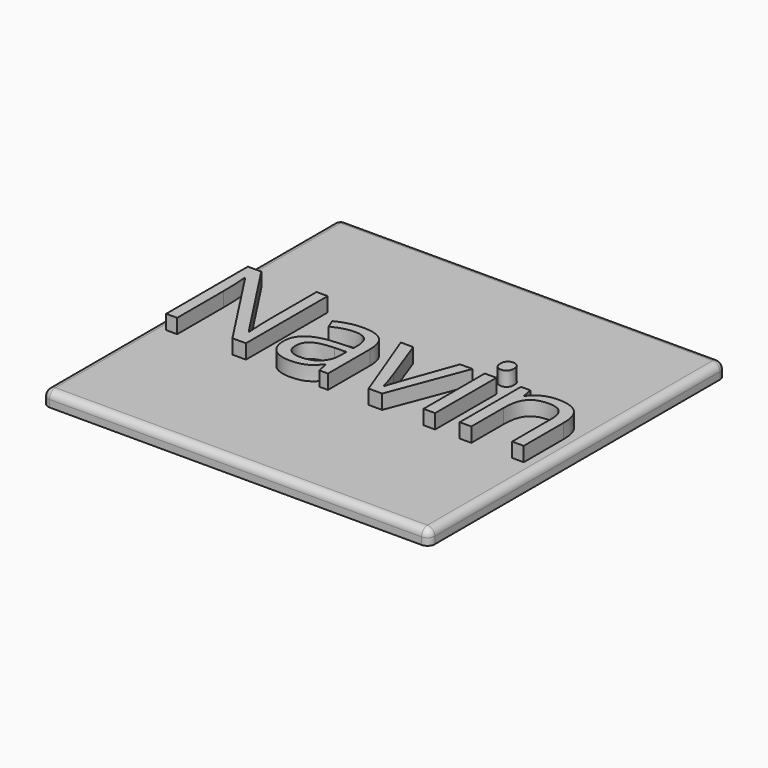
from build123d import *

# Parameters (mm, degrees)
F0_W         = 133.965395391
F0_H         = 128.5353191197
F1_DEPTH     = 5
F2_TEXT_SIZE = 49.5665770638
F3_DEPTH     = 5
F4_R         = 2.54
F5_R         = 2.54
F6_R         = 2.54
F7_R         = 2.54


# Not quite as in the source:
# - Text() gives the source's letters only with a copy of the font that has no kerning and outlines rounded to 1/6400 em; it was checked with that copy


with BuildPart() as f1:
    # F0 (on Top) → F1 (new body)
    with BuildSketch(Plane.XY):
        with Locations((-2.9858388007, 4.3018888682)):
            Rectangle(F0_W, F0_H)
    extrude(amount=F1_DEPTH)

    # F2 (on face) → F3 (join)
    with BuildSketch(Plane.XY.offset(5)):
        with Locations((-69.9685364962, -12.3775870944)):
            Text('Navin', F2_TEXT_SIZE, font='Open Sans', text_align=(TextAlign.LEFT, TextAlign.BOTTOM))
    extrude(amount=F3_DEPTH)

    # F4
    f4_edges = [f1.edges().sort_by_distance(p)[0] for p in [
        (-2.985839, -59.965771, 5),
    ]]
    fillet(f4_edges, radius=F4_R)

    # F5
    f5_edges = [f1.edges().sort_by_distance(p)[0] for p in [
        (63.996859, 5.571889, 5),
    ]]
    fillet(f5_edges, radius=F5_R)

    # F6
    f6_edges = [f1.edges().sort_by_distance(p)[0] for p in [
        (-69.968536, 5.571889, 5),
    ]]
    fillet(f6_edges, radius=F6_R)

    # F7
    f7_edges = [f1.edges().sort_by_distance(p)[0] for p in [
        (-2.985839, 68.569548, 5),
    ]]
    fillet(f7_edges, radius=F7_R)


solid = f1.part
